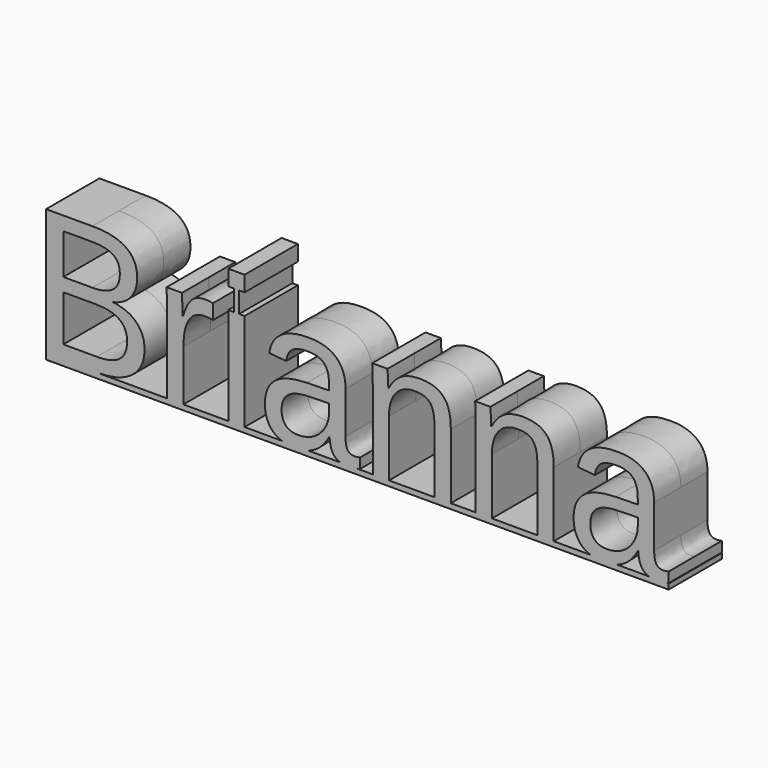
from build123d import *

# Parameters (mm, degrees)
F0_TEXT_SIZE = 35.2777777778
F1_DEPTH     = 6.35
F2_W         = 118.6931857639
F2_H         = 12.7
F3_DEPTH     = 1
F4_W         = 1
F4_H         = 3.9632378472
F5_DEPTH     = 12.7


# Not quite as in the source:
# - Text() gives the source's letters only with a copy of the font that has no kerning and outlines rounded to 1/6400 em; it was checked with that copy


with BuildPart() as f1:
    # F0 (on Front) → F1 (new body, symmetric)
    with BuildSketch(Plane.XZ):
        with Locations((-62.0172309028, 0)):
            Text('Brianna', F0_TEXT_SIZE, font='Arimo', text_align=(TextAlign.LEFT, TextAlign.BOTTOM))
    extrude(amount=F1_DEPTH, both=True)

    # F2 (on Top) → F3 (join)
    with BuildSketch(Plane.XY):
        with Locations((0.2232421875, 0)):
            Rectangle(F2_W, F2_H)
    extrude(amount=-F3_DEPTH)

    # F4 (on face) → F5 (join, through all)
    with BuildSketch(Plane.XZ.offset(6.35)):
        with Locations((-22.8285807292, 20.6182074653)):
            Rectangle(F4_W, F4_H)
    extrude(amount=-F5_DEPTH)


solid = f1.part
